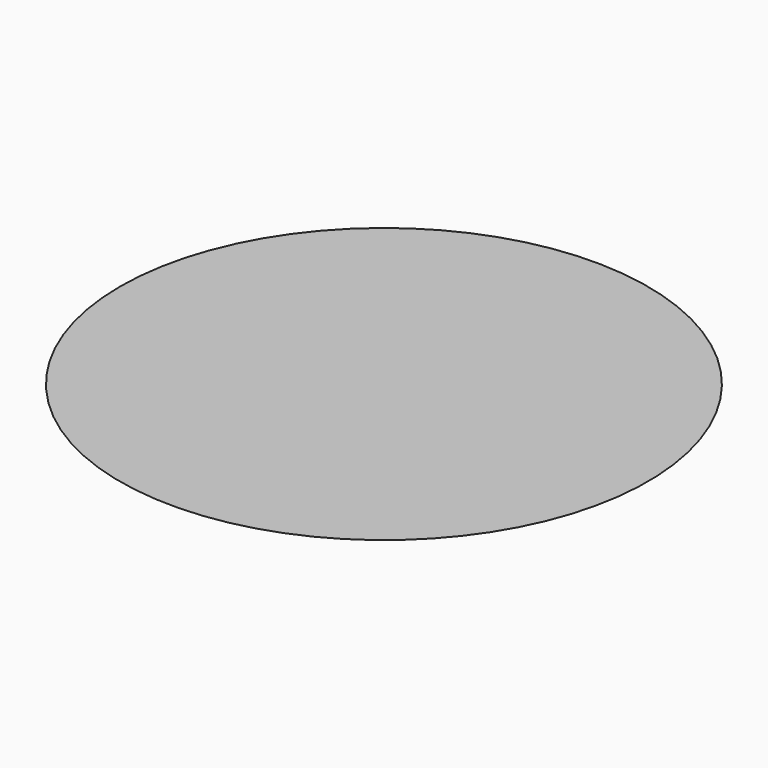
from build123d import *


with BuildPart() as f1:
    # F0 (on Front) → F1 (revolve)
    with BuildSketch(Plane.XZ):
        with BuildLine():
            ThreePointArc((-0.1678042017, 0.0084215911), (-0.084007698, 0.0021067218), (0, 0))
            Line((0, 0), (0, 0.0084215911))
            Line((0, 0.0084215911), (-0.1678042017, 0.0084215911))
        make_face()
    revolve(axis=Axis((0, 0, 1206.0346497539), (0, 0, 1)))


solid = f1.part
